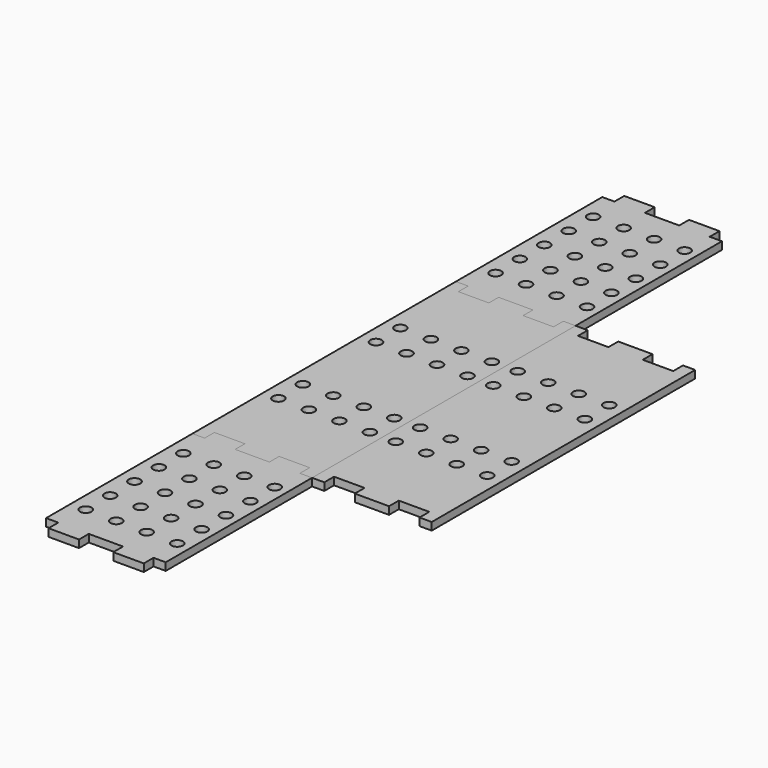
from build123d import *

# Parameters (mm, degrees)
F0_R     = 2.38125
F1_DEPTH = 3.175
F2_DEPTH = 3.175
F3_DEPTH = 3.175
F4_DEPTH = 3.175


# Not quite as in the source:
# - a length typed as a fraction of an inch, garbled in the dataset ("3 / 203.2 mm" for 3/8 in), is restored


with BuildPart() as f1:
    # F0 (on Top) → F1 (new body)
    with BuildSketch(Plane.XY):
        Polygon((23.1566016102, 68.58), (18.0766016102, 68.58), (18.0766016102, 38.1), (18.0766016102, -38.1), (18.0766016102, -68.58), (23.1566016102, -68.58), (23.1566016102, -63.5), (35.8566016102, -63.5), (35.8566016102, -68.58), (50.1232032204, -68.58), (50.1232032204, -63.5), (62.8232032204, -63.5), (62.8232032204, -68.58), (67.9032032204, -68.58), (67.9032032204, -38.1), (67.9032032204, 38.1), (67.9032032204, 68.58), (62.8232032204, 68.58), (62.8232032204, 63.5), (50.1232032204, 63.5), (50.1232032204, 68.58), (35.8566016102, 68.58), (35.8566016102, 63.5), (23.1566016102, 63.5), align=None)
        with Locations((23.4532032204, -31.75)):
            Circle(F0_R, mode=Mode.SUBTRACT)
        with Locations((23.4532032204, -19.05)):
            Circle(F0_R, mode=Mode.SUBTRACT)
        with Locations((36.1532032204, -31.75)):
            Circle(F0_R, mode=Mode.SUBTRACT)
        with Locations((36.1532032204, -19.05)):
            Circle(F0_R, mode=Mode.SUBTRACT)
        with Locations((48.8532032204, -31.75)):
            Circle(F0_R, mode=Mode.SUBTRACT)
        with Locations((48.8532032204, -19.05)):
            Circle(F0_R, mode=Mode.SUBTRACT)
        with Locations((61.5532032204, -31.75)):
            Circle(F0_R, mode=Mode.SUBTRACT)
        with Locations((61.5532032204, -19.05)):
            Circle(F0_R, mode=Mode.SUBTRACT)
        with Locations((23.4532032204, 19.05)):
            Circle(F0_R, mode=Mode.SUBTRACT)
        with Locations((23.4532032204, 31.75)):
            Circle(F0_R, mode=Mode.SUBTRACT)
        with Locations((36.1532032204, 19.05)):
            Circle(F0_R, mode=Mode.SUBTRACT)
        with Locations((36.1532032204, 31.75)):
            Circle(F0_R, mode=Mode.SUBTRACT)
        with Locations((48.8532032204, 19.05)):
            Circle(F0_R, mode=Mode.SUBTRACT)
        with Locations((48.8532032204, 31.75)):
            Circle(F0_R, mode=Mode.SUBTRACT)
        with Locations((61.5532032204, 19.05)):
            Circle(F0_R, mode=Mode.SUBTRACT)
        with Locations((61.5532032204, 31.75)):
            Circle(F0_R, mode=Mode.SUBTRACT)
    extrude(amount=F1_DEPTH)


with BuildPart() as f2:
    # F0 (on Top) → F2 (new body)
    with BuildSketch(Plane.XY):
        Polygon((-31.75, 68.58), (-31.75, 38.1), (-31.75, -38.1), (-31.75, -68.58), (-26.67, -68.58), (-26.67, -63.5), (-13.97, -63.5), (-13.97, -68.58), (0.2966016102, -68.58), (0.2966016102, -63.5), (12.9966016102, -63.5), (12.9966016102, -68.58), (18.0766016102, -68.58), (18.0766016102, -38.1), (18.0766016102, 38.1), (18.0766016102, 68.58), (12.9966016102, 68.58), (12.9966016102, 63.5), (0.2966016102, 63.5), (0.2966016102, 68.58), (-13.97, 68.58), (-13.97, 63.5), (-26.67, 63.5), (-26.67, 68.58), align=None)
        with Locations((-25.4, -31.75)):
            Circle(F0_R, mode=Mode.SUBTRACT)
        with Locations((-25.4, -19.05)):
            Circle(F0_R, mode=Mode.SUBTRACT)
        with Locations((-12.7, -31.75)):
            Circle(F0_R, mode=Mode.SUBTRACT)
        with Locations((-12.7, -19.05)):
            Circle(F0_R, mode=Mode.SUBTRACT)
        with Locations((0, -31.75)):
            Circle(F0_R, mode=Mode.SUBTRACT)
        with Locations((0, -19.05)):
            Circle(F0_R, mode=Mode.SUBTRACT)
        with Locations((12.7, -31.75)):
            Circle(F0_R, mode=Mode.SUBTRACT)
        with Locations((12.7, -19.05)):
            Circle(F0_R, mode=Mode.SUBTRACT)
        with Locations((-25.4, 19.05)):
            Circle(F0_R, mode=Mode.SUBTRACT)
        with Locations((-25.4, 31.75)):
            Circle(F0_R, mode=Mode.SUBTRACT)
        with Locations((-12.7, 19.05)):
            Circle(F0_R, mode=Mode.SUBTRACT)
        with Locations((-12.7, 31.75)):
            Circle(F0_R, mode=Mode.SUBTRACT)
        with Locations((0, 19.05)):
            Circle(F0_R, mode=Mode.SUBTRACT)
        with Locations((0, 31.75)):
            Circle(F0_R, mode=Mode.SUBTRACT)
        with Locations((12.7, 19.05)):
            Circle(F0_R, mode=Mode.SUBTRACT)
        with Locations((12.7, 31.75)):
            Circle(F0_R, mode=Mode.SUBTRACT)
    extrude(amount=F2_DEPTH)


with BuildPart() as f3:
    # F0 (on Top) → F3 (new body)
    with BuildSketch(Plane.XY):
        Polygon((-26.67, -68.58), (-31.75, -68.58), (-31.75, -144.78), (-26.67, -144.78), (-26.67, -149.86), (-13.97, -149.86), (-13.97, -144.78), (0.2966016102, -144.78), (0.2966016102, -149.86), (12.9966016102, -149.86), (12.9966016102, -144.78), (18.0766016102, -144.78), (18.0766016102, -68.58), (12.9966016102, -68.58), (12.9966016102, -63.5), (0.2966016102, -63.5), (0.2966016102, -68.58), (-13.97, -68.58), (-13.97, -63.5), (-26.67, -63.5), align=None)
        with Locations((-25.4, -132.08)):
            Circle(F0_R, mode=Mode.SUBTRACT)
        with Locations((-25.4, -119.38)):
            Circle(F0_R, mode=Mode.SUBTRACT)
        with Locations((-12.7, -132.08)):
            Circle(F0_R, mode=Mode.SUBTRACT)
        with Locations((-12.7, -119.38)):
            Circle(F0_R, mode=Mode.SUBTRACT)
        with Locations((-25.4, -106.68)):
            Circle(F0_R, mode=Mode.SUBTRACT)
        with Locations((-25.4, -93.98)):
            Circle(F0_R, mode=Mode.SUBTRACT)
        with Locations((-25.4, -81.28)):
            Circle(F0_R, mode=Mode.SUBTRACT)
        with Locations((-12.7, -106.68)):
            Circle(F0_R, mode=Mode.SUBTRACT)
        with Locations((-12.7, -93.98)):
            Circle(F0_R, mode=Mode.SUBTRACT)
        with Locations((-12.7, -81.28)):
            Circle(F0_R, mode=Mode.SUBTRACT)
        with Locations((0, -132.08)):
            Circle(F0_R, mode=Mode.SUBTRACT)
        with Locations((0, -119.38)):
            Circle(F0_R, mode=Mode.SUBTRACT)
        with Locations((12.7, -132.08)):
            Circle(F0_R, mode=Mode.SUBTRACT)
        with Locations((12.7, -119.38)):
            Circle(F0_R, mode=Mode.SUBTRACT)
        with Locations((0, -106.68)):
            Circle(F0_R, mode=Mode.SUBTRACT)
        with Locations((0, -93.98)):
            Circle(F0_R, mode=Mode.SUBTRACT)
        with Locations((0, -81.28)):
            Circle(F0_R, mode=Mode.SUBTRACT)
        with Locations((12.7, -106.68)):
            Circle(F0_R, mode=Mode.SUBTRACT)
        with Locations((12.7, -93.98)):
            Circle(F0_R, mode=Mode.SUBTRACT)
        with Locations((12.7, -81.28)):
            Circle(F0_R, mode=Mode.SUBTRACT)
    extrude(amount=F3_DEPTH)


with BuildPart() as f4:
    # F0 (on Top) → F4 (new body)
    with BuildSketch(Plane.XY):
        Polygon((-31.75, 144.78), (-31.75, 68.58), (-26.67, 68.58), (-26.67, 63.5), (-13.97, 63.5), (-13.97, 68.58), (0.2966016102, 68.58), (0.2966016102, 63.5), (12.9966016102, 63.5), (12.9966016102, 68.58), (18.0766016102, 68.58), (18.0766016102, 144.78), (12.9966016102, 144.78), (12.9966016102, 149.86), (0.2966016102, 149.86), (0.2966016102, 144.78), (-13.97, 144.78), (-13.97, 149.86), (-26.67, 149.86), (-26.67, 144.78), align=None)
        with Locations((-25.4, 81.28)):
            Circle(F0_R, mode=Mode.SUBTRACT)
        with Locations((-25.4, 93.98)):
            Circle(F0_R, mode=Mode.SUBTRACT)
        with Locations((-25.4, 106.68)):
            Circle(F0_R, mode=Mode.SUBTRACT)
        with Locations((-12.7, 81.28)):
            Circle(F0_R, mode=Mode.SUBTRACT)
        with Locations((-12.7, 93.98)):
            Circle(F0_R, mode=Mode.SUBTRACT)
        with Locations((-12.7, 106.68)):
            Circle(F0_R, mode=Mode.SUBTRACT)
        with Locations((-25.4, 119.38)):
            Circle(F0_R, mode=Mode.SUBTRACT)
        with Locations((-25.4, 132.08)):
            Circle(F0_R, mode=Mode.SUBTRACT)
        with Locations((-12.7, 119.38)):
            Circle(F0_R, mode=Mode.SUBTRACT)
        with Locations((-12.7, 132.08)):
            Circle(F0_R, mode=Mode.SUBTRACT)
        with Locations((0, 81.28)):
            Circle(F0_R, mode=Mode.SUBTRACT)
        with Locations((0, 93.98)):
            Circle(F0_R, mode=Mode.SUBTRACT)
        with Locations((0, 106.68)):
            Circle(F0_R, mode=Mode.SUBTRACT)
        with Locations((12.7, 81.28)):
            Circle(F0_R, mode=Mode.SUBTRACT)
        with Locations((12.7, 93.98)):
            Circle(F0_R, mode=Mode.SUBTRACT)
        with Locations((12.7, 106.68)):
            Circle(F0_R, mode=Mode.SUBTRACT)
        with Locations((0, 119.38)):
            Circle(F0_R, mode=Mode.SUBTRACT)
        with Locations((0, 132.08)):
            Circle(F0_R, mode=Mode.SUBTRACT)
        with Locations((12.7, 119.38)):
            Circle(F0_R, mode=Mode.SUBTRACT)
        with Locations((12.7, 132.08)):
            Circle(F0_R, mode=Mode.SUBTRACT)
    extrude(amount=F4_DEPTH)


solid = Compound([f1.part, f2.part, f3.part, f4.part])
